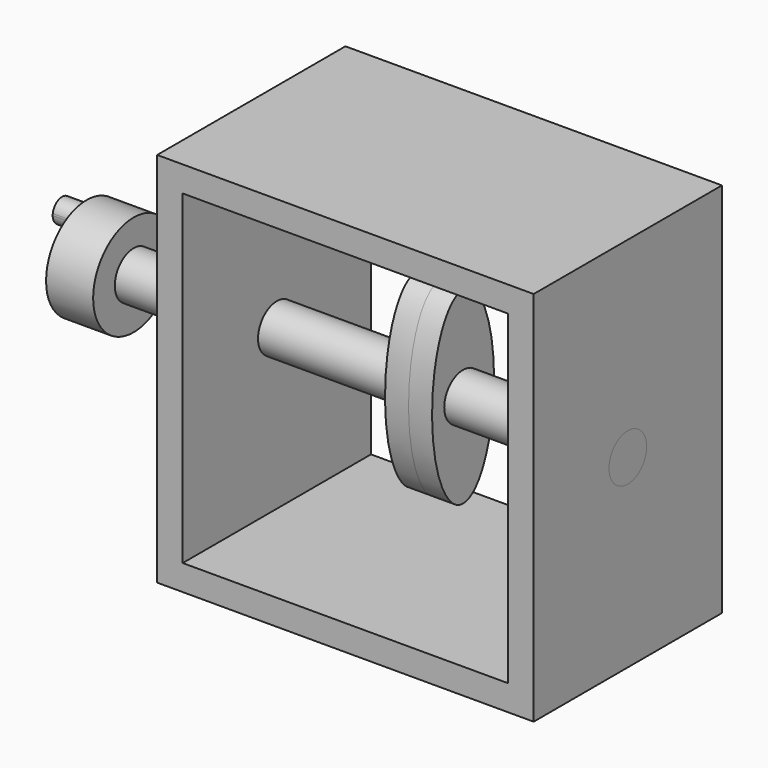
from build123d import *

# Parameters (mm, degrees)
F0_W          = 101.6
F0_H          = 101.6
F1_DEPTH      = 31.75
F2_W          = 87.7997364508
F2_H          = 87.7997364508
F3_DEPTH      = 101.6
F4_R          = 6.35
F5_DEPTH      = 44.45
F5_DEPTH_BACK = 101.6
F9_DEPTH      = 6.35
F11_R         = 13.6518424836
F11_R_2       = 6.35
F12_DEPTH     = 12.7
F14_DEPTH     = 12.7


# Not quite as in the source:
# - the program builds the solid bodies; features that only make, move or delete a surface that nothing else refers to are left out


with BuildPart() as f1:
    # F0 (on Front) → F1 (new body, symmetric)
    with BuildSketch(Plane.XZ):
        with Locations((3.7253e-06, 0.921211595)):
            Rectangle(F0_W, F0_H)
    extrude(amount=F1_DEPTH, both=True)

    # F2 (on face) → F3 (cut)
    with BuildSketch(Plane.XZ.offset(31.75)):
        with Locations((3.7253e-06, 0.921211595)):
            Rectangle(F2_W, F2_H)
    extrude(amount=-F3_DEPTH, mode=Mode.SUBTRACT)


with BuildPart() as f5:
    # F4 (on face) → F5 (new body, two sides)
    with BuildSketch(Plane(origin=(-50.7999962747, 0, 0), x_dir=(0, -1, 0), z_dir=(-1, 0, 0))) as f5_sk:
        Circle(F4_R)
    extrude(amount=F5_DEPTH)
    extrude(f5_sk.sketch, amount=-F5_DEPTH_BACK)

    # F11 (on face) → F12 (join)
    with BuildSketch(Plane(origin=(-95.2499962747, 0, 0), x_dir=(0, -1, 0), z_dir=(-1, 0, 0))):
        Circle(F11_R)
        Circle(F11_R_2, mode=Mode.SUBTRACT)
    extrude(amount=-F12_DEPTH)

    # F13 (on face) → F14 (join)
    with BuildSketch(Plane(origin=(-95.2499962747, 0, 0), x_dir=(0, -1, 0), z_dir=(-1, 0, 0))):
        with BuildLine():
            ThreePointArc((-6.2429233087, 1.1612099561), (-5.6174872871, 2.9607999898), (-4.486384138, 4.4938688639))
            ThreePointArc((-4.486384138, 4.4938688639), (-10.434456191, 5.4996720429), (-6.2429233087, 1.1612099561))
        make_face()
        with BuildLine():
            ThreePointArc((-6.2429233087, 1.1612099561), (-4.9358258553, 2.332519374), (-4.4507125475, 4.019272048))
            ThreePointArc((-4.4507125475, 4.019272048), (-4.4596430046, 4.257239798), (-4.486384138, 4.4938688639))
            ThreePointArc((-4.486384138, 4.4938688639), (-5.6174872871, 2.9607999898), (-6.2429233087, 1.1612099561))
        make_face()
    extrude(amount=F14_DEPTH)


with BuildPart() as f9:
    # F8 (on Right) → F9 (new body, symmetric)
    with BuildSketch(Plane.YZ):
        with BuildLine():
            add(Edge.make_bspline(
                [(0, 25.4), (-18.1230958021, 25.4), (-9.0615479011, -12.7), (0, -50.8), (9.0615479011, -12.7), (18.1230958021, 25.4), (0, 25.4)],
                knots=[0, 0, 0, 2.0943951024, 2.0943951024, 4.1887902048, 4.1887902048, 6.2831853072, 6.2831853072, 6.2831853072], degree=2, weights=[1, 0.5, 1, 0.5, 1, 0.5, 1]))
        make_face()
    extrude(amount=F9_DEPTH, both=True)


solid = Compound([f1.part, f5.part, f9.part])
